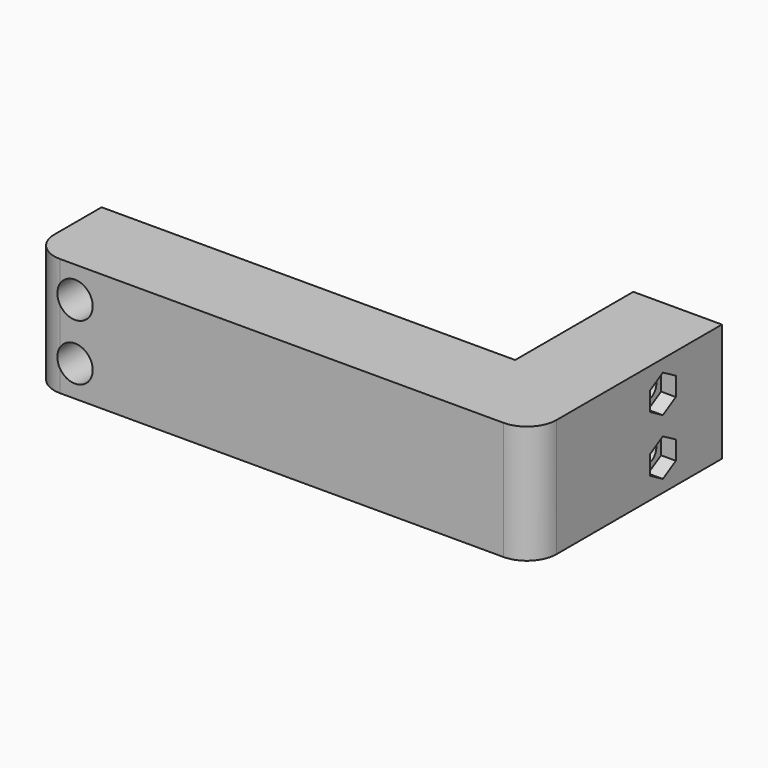
from build123d import *

# Parameters (mm, degrees)
F1_DEPTH    = 20
F2_R        = 1.75
F3_DEPTH    = 40.001
F4_R        = 3
F5_DEPTH    = 7.5
F6_R        = 1.75
F7_DEPTH    = 15.001
F8_T1_DEPTH = 45
F10_DEPTH   = 2.5


# Not quite as in the source:
# - a fillet or chamfer that OpenCascade refuses, or shapes differently, is made with other operations: its cross-section is extruded or revolved along the edge and cut away or added


with BuildPart() as f1:
    # F0 (on Top) → F1 (new body)
    with BuildSketch(Plane.XY):
        Polygon((0, 15), (0, 0), (85, 0), (85, 40), (70, 40), (70, 15), align=None)
    extrude(amount=F1_DEPTH)

    # F2 (on face) → F3 (cut, through all)
    with BuildSketch(Plane.XZ):
        with Locations((7.5, 14.75)):
            Circle(F2_R)
        with Locations((7.5, 5.25)):
            Circle(F2_R)
    extrude(amount=-F3_DEPTH, mode=Mode.SUBTRACT)

    # F4 (on face) → F5 (cut)
    with BuildSketch(Plane.XZ):
        with Locations((7.5, 14.75)):
            Circle(F4_R)
        with Locations((7.5, 5.25)):
            Circle(F4_R)
    extrude(amount=-F5_DEPTH, mode=Mode.SUBTRACT)

    # F6 (on face) → F7 (cut, through all)
    with BuildSketch(Plane(origin=(70, 0, 0), x_dir=(0, -1, 0), z_dir=(-1, 0, 0))):
        with Locations((-27.5, 14.75)):
            Circle(F6_R)
        with Locations((-27.5, 5.25)):
            Circle(F6_R)
    extrude(amount=-F7_DEPTH, mode=Mode.SUBTRACT)

    # F8: fillet of radius 5 on 2 edges, made by hand

    # F8_s2 → F8_t1 (cut)
    with BuildSketch(Plane.XY.offset(-12.5)):
        with BuildLine():
            ThreePointArc((80, 0), (83.5355339059, 1.4644660941), (85, 5))
            Line((85, 5), (85, 0))
            Line((85, 0), (80, 0))
        make_face()
        with BuildLine():
            ThreePointArc((0, 5), (1.4644660941, 1.4644660941), (5, 0))
            Line((5, 0), (0, 0))
            Line((0, 0), (0, 5))
        make_face()
    extrude(amount=F8_T1_DEPTH, mode=Mode.SUBTRACT)

    # F9 (on face) → F10 (cut)
    with BuildSketch(Plane.YZ.offset(85)):
        Polygon((27.5, 11.5745735195), (30.25, 13.1622867597), (30.25, 16.3377132403), (27.5, 17.9254264805), (24.75, 16.3377132403), (24.75, 13.1622867597), align=None)
        Polygon((30.25, 6.8377132403), (27.5, 8.4254264805), (24.75, 6.8377132403), (24.75, 3.6622867597), (27.5, 2.0745735195), (30.25, 3.6622867597), align=None)
    extrude(amount=-F10_DEPTH, mode=Mode.SUBTRACT)


solid = f1.part
